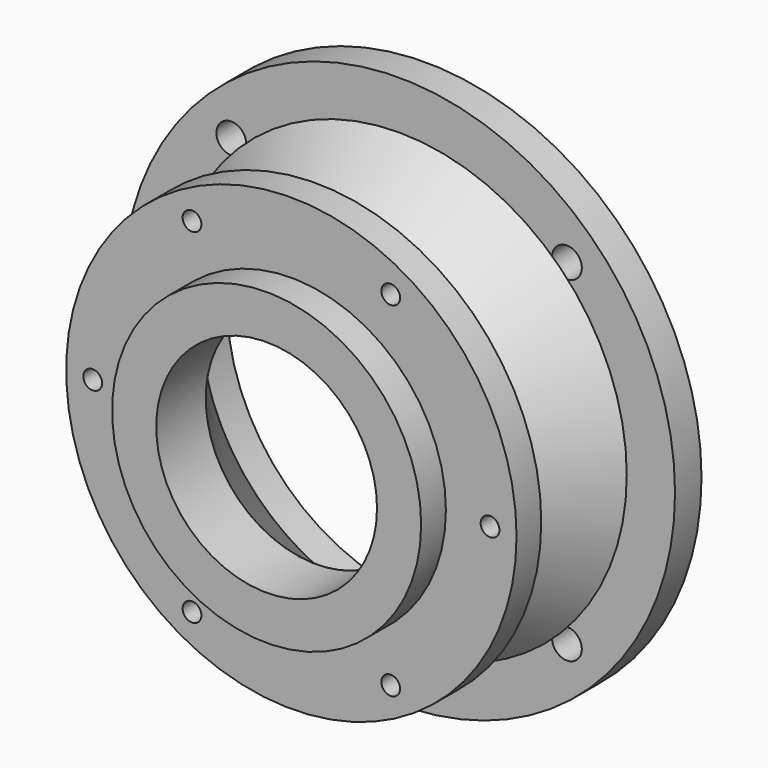
from build123d import *

# Parameters (mm, degrees)
F0_R             = 125
F1_DEPTH         = 15
F4_R             = 102
F5_DEPTH         = 14
F6_R             = 70
F7_DEPTH         = 14
F9_D             = 8.5
F9_DEPTH         = 19.5
F9_TIP           = 2.5536576309
F9_COPIES_COUNT  = 6
F2_R             = 90
F10_DEPTH        = 25
F12_D            = 13.5
F12_DEPTH        = 20
F12_TIP          = 4.0558091784
F12_COPIES_COUNT = 4
F13_R            = 50
F14_DEPTH        = 90.001


# Not quite as in the source:
# - a pattern or mirror of a feature is missing from the dataset's text; its kind, count and spacing are read off the source's solid


with BuildPart() as f1:
    # F0 (on Front) → F1 (new body)
    with BuildSketch(Plane.XZ):
        Circle(F0_R)
    extrude(amount=F1_DEPTH)

    # F2 (on face) → F10 (cut)
    with BuildSketch(Plane.XZ.offset(15)):
        Circle(F2_R)
    extrude(amount=-F10_DEPTH, mode=Mode.SUBTRACT)

    # F12
    with Locations(Plane.XZ.offset(15)):
        with Locations((76.0139789776, 76.0139789776)):
            f12 = Hole(F12_D / 2, depth=F12_DEPTH)
            with Locations((0, 0, -(F12_DEPTH + F12_TIP / 2))):  # 118° drill point
                Cone(0, F12_D / 2, F12_TIP, mode=Mode.SUBTRACT)

    # F12_copies: F12 ×4 about axis
    f12_copies_axis = Axis((0, 0, 0), (0, 1, 0))
    for i in range(1, F12_COPIES_COUNT):
        add(f12.rotate(f12_copies_axis, i * 360 / F12_COPIES_COUNT), mode=Mode.SUBTRACT)


with BuildPart() as f5:
    # F4 (on offset) → F5 (new body)
    with BuildSketch(Plane.XZ.offset(62)):
        Circle(F4_R)
    extrude(amount=F5_DEPTH)

    # F6 (on face) → F7 (join)
    with BuildSketch(Plane.XZ.offset(76)):
        Circle(F6_R)
    extrude(amount=F7_DEPTH)

    # F9
    with Locations(Plane.XZ.offset(76)):
        with Locations((45, 77.9422863406)):
            f9 = Hole(F9_D / 2, depth=F9_DEPTH)
            with Locations((0, 0, -(F9_DEPTH + F9_TIP / 2))):  # 118° drill point
                Cone(0, F9_D / 2, F9_TIP, mode=Mode.SUBTRACT)

    # F9_copies: F9 ×6 about axis
    f9_copies_axis = Axis((0, 0, 0), (0, 1, 0))
    for i in range(1, F9_COPIES_COUNT):
        add(f9.rotate(f9_copies_axis, i * 360 / F9_COPIES_COUNT), mode=Mode.SUBTRACT)

    # F13 (on face) → F14 (cut, through all)
    with BuildSketch(Plane.XZ.offset(90)):
        Circle(F13_R)
    extrude(amount=-F14_DEPTH, mode=Mode.SUBTRACT)


with BuildPart() as f16:
    # F15 (on Right) → F16 (revolve)
    with BuildSketch(Plane.YZ):
        Polygon((-62, 63.131297127), (-62, 50), (-15, 90), (-15, 103.131297127), align=None)
    revolve(axis=Axis((0, -76, 0), (0, -1, 0)))


solid = Compound([f1.part, f5.part, f16.part])
